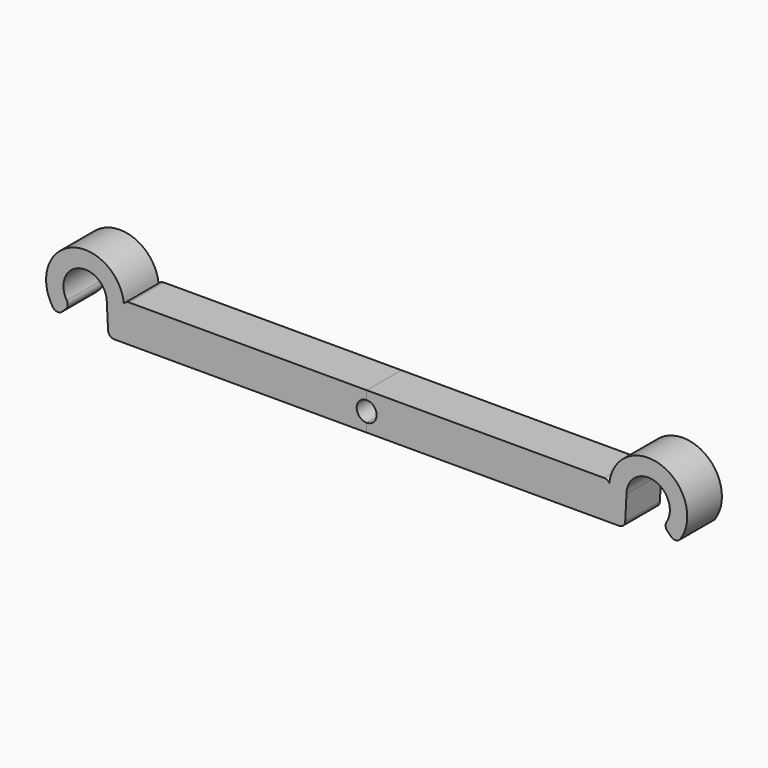
from build123d import *
from build123d import SkipClean  # not in build123d's __all__

# Parameters (mm, degrees)
F1_DEPTH    = 5
F2_T1_DEPTH = 8.0563067351
F2_T3_DEPTH = 8.3213759835
F2_T5_DEPTH = 8.112494996
F2_T7_DEPTH = 9.1625838734


# Not quite as in the source:
# - a fillet or chamfer that OpenCascade refuses, or shapes differently, is made with other operations: its cross-section is extruded or revolved along the edge and cut away or added


with BuildPart() as f1:
    # F0 (on Front) → F1 (new body)
    with BuildSketch(Plane.XZ):
        with BuildLine():
            Line((0, -1), (0, 0))
            Line((0, 0), (-27.9919262234, 0))
            Line((-27.9919262234, 0), (-27.9746514708, -0.3296219153))
            ThreePointArc((-27.9746514708, -0.3296219153), (-34.3872999356, 3.2616337796), (-35.6319805153, -3.9819805153))
            Line((-35.6319805153, -3.9819805153), (-34.217766953, -2.567766953))
            ThreePointArc((-34.217766953, -2.567766953), (-33.4067085809, 1.5096988313), (-29.95, -0.8))
            Line((-29.95, -0.8), (-29.7665727725, -4.3))
            Line((-29.7665727725, -4.3), (0, -4.3))
            Line((0, -4.3), (0, -3.3))
            ThreePointArc((0, -3.3), (-1.15, -2.15), (0, -1))
        make_face()
        with BuildLine():
            Line((-27.95, -0.8), (-27.9746514708, -0.3296219153))
            ThreePointArc((-27.9746514708, -0.3296219153), (-27.9561670936, -0.5644881969), (-27.95, -0.8))
        make_face(mode=Mode.SUBTRACT)
        with BuildLine():
            ThreePointArc((-27.95, -0.8), (-27.9561670936, -0.5644881969), (-27.9746514708, -0.3296219153))
            Line((-27.9746514708, -0.3296219153), (-27.95, -0.8))
        make_face()
    extrude(amount=F1_DEPTH)

    # F2: fillet of radius 0.7 on 4 edges, made by hand

    # F2_s2 → F2_t1 (cut)
    with BuildSketch(Plane.XZ.offset(-1.5281533676)):
        with BuildLine():
            ThreePointArc((-27.3806648764, 0), (-27.7203230433, -0.0879278395), (-27.9746514708, -0.3296219153))
            Line((-27.9746514708, -0.3296219153), (-27.9919262234, 0))
            Line((-27.9919262234, 0), (-27.3806648764, 0))
        make_face()
    extrude(amount=F2_T1_DEPTH, mode=Mode.SUBTRACT)

    # F2_s4 → F2_t3 (cut)
    with BuildSketch(Plane.XZ.offset(-1.6606879918)):
        with BuildLine():
            ThreePointArc((-29.1022975758, -4.3), (-29.5841457788, -4.1077620597), (-29.8013382501, -3.6366351694))
            Line((-29.8013382501, -3.6366351694), (-29.7665727725, -4.3))
            Line((-29.7665727725, -4.3), (-29.1022975758, -4.3))
        make_face()
    extrude(amount=F2_T3_DEPTH, mode=Mode.SUBTRACT)

    # F2_s6 → F2_t5 (cut)
    with BuildSketch(Plane.XZ.offset(-1.556247498)):
        with BuildLine():
            ThreePointArc((-34.6579402166, -3.0079402166), (-34.4571662087, -2.5899957909), (-34.5616523152, -2.1382542732))
            ThreePointArc((-34.5616523152, -2.1382542732), (-34.4015618745, -2.3625), (-34.217766953, -2.567766953))
            Line((-34.217766953, -2.567766953), (-34.6579402166, -3.0079402166))
        make_face()
    extrude(amount=F2_T5_DEPTH, mode=Mode.SUBTRACT)

    # F2_s8 → F2_t7 (cut)
    with BuildSketch(Plane.XZ.offset(-2.0812919367)):
        with BuildLine():
            ThreePointArc((-36.1636809848, -3.3413723739), (-35.6507485808, -3.6430465403), (-35.0910225292, -3.4410225292))
            Line((-35.0910225292, -3.4410225292), (-35.6319805153, -3.9819805153))
            ThreePointArc((-35.6319805153, -3.9819805153), (-35.9126769383, -3.6739986815), (-36.1636809848, -3.3413723739))
        make_face()
    extrude(amount=F2_T7_DEPTH, mode=Mode.SUBTRACT)

    # F3: F1 across plane


with BuildPart() as f1_1:
    add(f1.part, clean=False)
    with SkipClean():  # cleaning this boolean's faces spoils the solid; the shape is the same uncleaned
        add(f1.part.mirror(Plane.YZ), clean=False)


solid = f1_1.part
